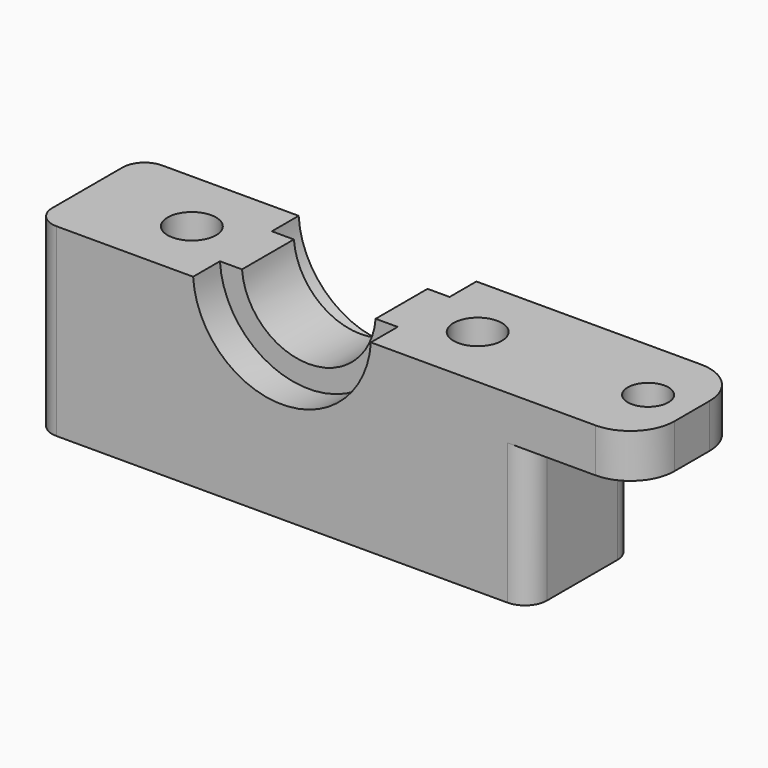
from build123d import *

# Parameters (mm, degrees)
F0_W      = 45
F0_H      = 12
F0_R      = 2.2
F1_DEPTH  = 16.8
F3_DEPTH  = 12.001
F4_R      = 8.1
F5_DEPTH  = 3.05
F6_R      = 8.1
F7_DEPTH  = 3.05
F8_R      = 4.5
F8_R_2    = 2.2
F9_DEPTH  = 9
F10_SIZE  = 2.29999
F11_R     = 2
F12_W     = 12
F12_H     = 12
F12_R     = 1.85
F13_DEPTH = 4
F14_R     = 4


# Not quite as in the source:
# - a fillet or chamfer is up to 0.001 mm smaller than in the source, because OpenCascade refuses the exact size


with BuildPart() as f1:
    # F0 (on Top) → F1 (new body)
    with BuildSketch(Plane.XY):
        Rectangle(F0_W, F0_H)
        with Locations((-13, 0)):
            Circle(F0_R, mode=Mode.SUBTRACT)
        with Locations((13, 0)):
            Circle(F0_R, mode=Mode.SUBTRACT)
    extrude(amount=F1_DEPTH)

    # F2 (on face) → F3 (cut, through all)
    with BuildSketch(Plane(origin=(0, 6, 0), x_dir=(-1, 0, 0), z_dir=(0, 1, 0))):
        with BuildLine():
            ThreePointArc((-6.0794736614, 16.8), (0, 11.2), (6.0794736614, 16.8))
            Line((6.0794736614, 16.8), (-6.0794736614, 16.8))
        make_face()
        with BuildLine():
            Line((-6.0794736614, 16.8), (6.0794736614, 16.8))
            ThreePointArc((6.0794736614, 16.8), (6.0948662551, 17.0497894234), (6.1, 17.3))
            ThreePointArc((6.1, 17.3), (-0.2502105766, 23.3948662551), (-6.0794736614, 16.8))
        make_face()
    extrude(amount=-F3_DEPTH, mode=Mode.SUBTRACT)

    # F4 (on face) → F5 (cut)
    with BuildSketch(Plane(origin=(0, 6, 0), x_dir=(-1, 0, 0), z_dir=(0, 1, 0))):
        with Locations((0, 17.3)):
            Circle(F4_R)
    extrude(amount=-F5_DEPTH, mode=Mode.SUBTRACT)

    # F6 (on face) → F7 (cut)
    with BuildSketch(Plane.XZ.offset(6)):
        with Locations((0, 17.3)):
            Circle(F6_R)
    extrude(amount=-F7_DEPTH, mode=Mode.SUBTRACT)

    # F8 (on face) → F9 (cut)
    with BuildSketch(Plane(origin=(0, 0, 0), x_dir=(1, 0, 0), z_dir=(0, 0, -1))):
        with Locations((-13, 0)):
            Circle(F8_R)
        with Locations((-13, 0)):
            Circle(F8_R_2, mode=Mode.SUBTRACT)
        with Locations((13, 0)):
            Circle(F8_R)
        with Locations((13, 0)):
            Circle(F8_R_2, mode=Mode.SUBTRACT)
    extrude(amount=-F9_DEPTH, mode=Mode.SUBTRACT)

    # F10 (size 2.3 in the source; OpenCascade refuses exactly that, so slightly less here)
    f10_edges = [f1.edges().sort_by_distance(p)[0] for p in [
        (-17.5, 0, 9),
        (8.5, 0, 9),
    ]]
    chamfer(f10_edges, length=F10_SIZE)

    # F11
    f11_edges = [f1.edges().sort_by_distance(p)[0] for p in [
        (22.5, -6, 8.4),
        (-22.5, -6, 8.4),
        (22.5, 6, 8.4),
        (-22.5, 6, 8.4),
    ]]
    fillet(f11_edges, radius=F11_R)

    # F12 (on face) → F13 (join)
    with BuildSketch(Plane.XY.offset(16.8)):
        with Locations((26.5, 0)):
            Rectangle(F12_W, F12_H)
        with Locations((28.5, 0)):
            Circle(F12_R, mode=Mode.SUBTRACT)
    extrude(amount=-F13_DEPTH)

    # F14
    f14_edges = [f1.edges().sort_by_distance(p)[0] for p in [
        (32.5, -6, 14.8),
        (32.5, 6, 14.8),
    ]]
    fillet(f14_edges, radius=F14_R)


solid = f1.part
